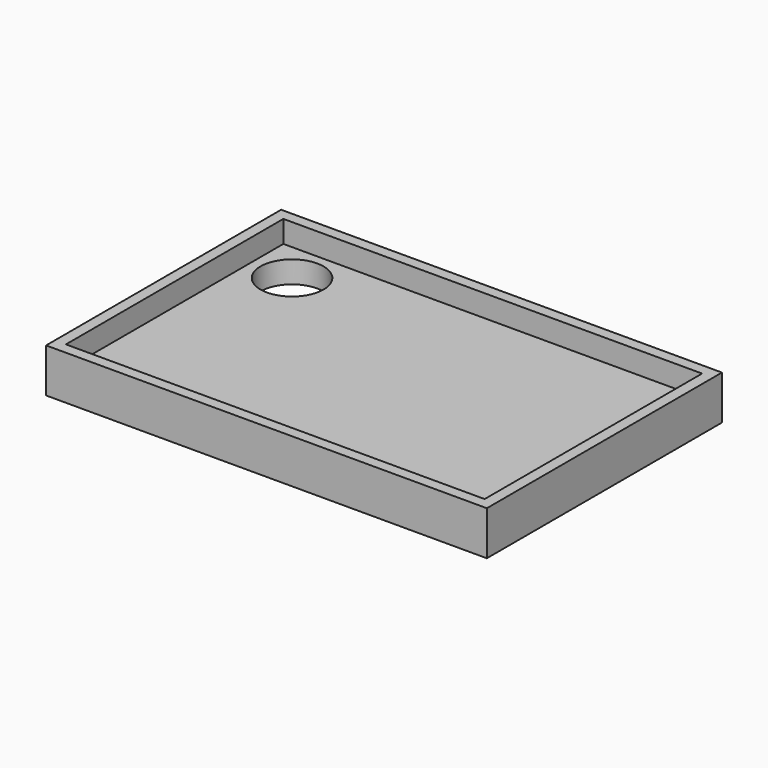
from build123d import *

# Parameters (mm, degrees)
F0_W     = 60
F0_H     = 40
F1_DEPTH = 3
F2_W     = 57
F2_H     = 37
F3_DEPTH = 3
F6_R     = 4.2845281604
F7_DEPTH = 6


# Not quite as in the source:
# - the program builds the solid bodies; features that only make, move or delete a surface that nothing else refers to are left out


with BuildPart() as f1:
    # F0 (on Top) → F1 (new body, symmetric)
    with BuildSketch(Plane.XY):
        Rectangle(F0_W, F0_H)
    extrude(amount=F1_DEPTH, both=True)

    # F2 (on face) → F3 (cut)
    with BuildSketch(Plane.XY.offset(3)):
        Rectangle(F2_W, F2_H)
    extrude(amount=-F3_DEPTH, mode=Mode.SUBTRACT)

    # F6 (on face) → F7 (cut)
    with BuildSketch(Plane.XY):
        with Locations((-22.8839740157, 12.9562756047)):
            Circle(F6_R)
    extrude(amount=-F7_DEPTH, mode=Mode.SUBTRACT)


solid = f1.part
